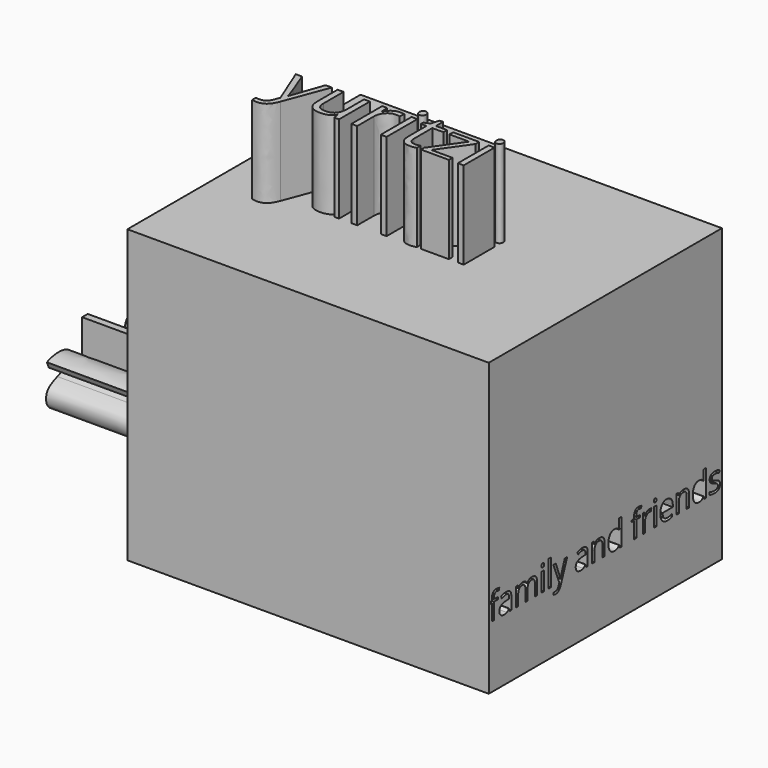
from build123d import *

# Parameters (mm, degrees)
F0_W         = 127
F0_H         = 127
F1_DEPTH     = 127
F2_TEXT_SIZE = 31.3097072419
F3_DEPTH     = 38.1
F4_TEXT_SIZE = 37.9493149618
F5_DEPTH     = 38.1
F6_TEXT_SIZE = 18.0097937116
F7_DEPTH     = 30.48
F8_W         = 127
F8_H         = 127
F8_W_2       = 1.2229891456
F8_H_2       = 8.0707857872
F8_H_3       = 11.4593376009
F9_DEPTH     = 30.48


# Not quite as in the source:
# - Text() gives the source's letters only with a copy of the font that has no kerning and outlines rounded to 1/6400 em; it was checked with that copy


with BuildPart() as f1:
    # F0 (on Front) → F1 (new body)
    with BuildSketch(Plane.XZ):
        with Locations((29.3806100488, 72.0371453315)):
            Rectangle(F0_W, F0_H)
    extrude(amount=F1_DEPTH)

    # F2 (on face) → F3 (join)
    with BuildSketch(Plane.XY.offset(135.5371453315)):
        with Locations((-15.0693899512, -75.8829892142)):
            Text('yuritzi', F2_TEXT_SIZE, font='Open Sans', text_align=(TextAlign.LEFT, TextAlign.BOTTOM))
    extrude(amount=F3_DEPTH)

    # F4 (on face) → F5 (join)
    with BuildSketch(Plane(origin=(-34.1193899512, 0, 0), x_dir=(0, -1, 0), z_dir=(-1, 0, 0))):
        with Locations((1.5054866672, 51.249936223)):
            Text('friends', F4_TEXT_SIZE, font='Open Sans', text_align=(TextAlign.LEFT, TextAlign.BOTTOM))
    extrude(amount=F5_DEPTH)

    # F6 (on face) → F7 (join)
    with BuildSketch(Plane(origin=(0, 0, 0), x_dir=(-1, 0, 0), z_dir=(0, 1, 0))):
        with Locations((-92.8806100488, 35.0644422385)):
            Text('happy holidays', F6_TEXT_SIZE, font='Open Sans', text_align=(TextAlign.LEFT, TextAlign.BOTTOM))
    extrude(amount=F7_DEPTH)

    # F8 (on face) → F9 (join)
    with BuildSketch(Plane.YZ.offset(92.8806100488)):
        with Locations((-63.5, 72.0371453315)):
            Rectangle(F8_W, F8_H)
        with BuildLine():
            Line((-114.7229798683, 35.6142357407), (-115.6302068838, 35.6142357407))
            Line((-115.6302068838, 35.6142357407), (-115.8729195658, 36.7641754382))
            Line((-115.8729195658, 36.7641754382), (-115.931830411, 36.7641754382))
            add(Edge.make_bspline(
                [(-115.931830411, 36.7641754382), (-116.5350774654, 36.0054037525), (-117.1347898692, 35.7355920817)],
                knots=[0, 0, 0, 1, 1, 1], degree=2))
            add(Edge.make_bspline(
                [(-117.1347898692, 35.7355920817), (-117.7345022729, 35.4657804109), (-118.634659987, 35.4657804109)],
                knots=[0, 0, 0, 1, 1, 1], degree=2))
            add(Edge.make_bspline(
                [(-118.634659987, 35.4657804109), (-119.8340847945, 35.4657804109), (-120.5150941646, 36.085522502)],
                knots=[0, 0, 0, 1, 1, 1], degree=2))
            add(Edge.make_bspline(
                [(-120.5150941646, 36.085522502), (-121.1961035347, 36.7052645931), (-121.1961035347, 37.8457785554)],
                knots=[0, 0, 0, 1, 1, 1], degree=2))
            add(Edge.make_bspline(
                [(-121.1961035347, 37.8457785554), (-121.1961035347, 40.2894004127), (-117.2867798497, 40.407222103)],
                knots=[0, 0, 0, 1, 1, 1], degree=2))
            Line((-117.2867798497, 40.407222103), (-115.9176918081, 40.4519943454))
            Line((-115.9176918081, 40.4519943454), (-115.9176918081, 40.9539147461))
            add(Edge.make_bspline(
                [(-115.9176918081, 40.9539147461), (-115.9176918081, 41.9035575701), (-116.3253548567, 42.355992861)],
                knots=[0, 0, 0, 1, 1, 1], degree=2))
            add(Edge.make_bspline(
                [(-116.3253548567, 42.355992861), (-116.7330179052, 42.8084281518), (-117.6331756193, 42.8084281518)],
                knots=[0, 0, 0, 1, 1, 1], degree=2))
            add(Edge.make_bspline(
                [(-117.6331756193, 42.8084281518), (-118.6417292884, 42.8084281518), (-119.9142035439, 42.1910424945)],
                knots=[0, 0, 0, 1, 1, 1], degree=2))
            Line((-119.9142035439, 42.1910424945), (-120.291232953, 43.1265467157))
            add(Edge.make_bspline(
                [(-120.291232953, 43.1265467157), (-119.6950551999, 43.4493781472), (-118.9845904073, 43.6331799841)],
                knots=[0, 0, 0, 1, 1, 1], degree=2))
            add(Edge.make_bspline(
                [(-118.9845904073, 43.6331799841), (-118.2741256146, 43.816981821), (-117.5577697375, 43.816981821)],
                knots=[0, 0, 0, 1, 1, 1], degree=2))
            add(Edge.make_bspline(
                [(-117.5577697375, 43.816981821), (-116.1156322479, 43.816981821), (-115.4193060581, 43.1772100425)],
                knots=[0, 0, 0, 1, 1, 1], degree=2))
            add(Edge.make_bspline(
                [(-115.4193060581, 43.1772100425), (-114.7229798683, 42.5374382641), (-114.7229798683, 41.1235779802)],
                knots=[0, 0, 0, 1, 1, 1], degree=2))
            Line((-114.7229798683, 41.1235779802), (-114.7229798683, 35.6142357407))
        make_face(mode=Mode.SUBTRACT)
        with BuildLine():
            Line((-100.6974858521, 35.6142357407), (-101.9181185639, 35.6142357407))
            Line((-101.9181185639, 35.6142357407), (-101.9181185639, 40.8643702615))
            add(Edge.make_bspline(
                [(-101.9181185639, 40.8643702615), (-101.9181185639, 41.8305081221), (-102.33049448, 42.3123988356)],
                knots=[0, 0, 0, 1, 1, 1], degree=2))
            add(Edge.make_bspline(
                [(-102.33049448, 42.3123988356), (-102.7428703961, 42.794289549), (-103.6123944707, 42.794289549)],
                knots=[0, 0, 0, 1, 1, 1], degree=2))
            add(Edge.make_bspline(
                [(-103.6123944707, 42.794289549), (-104.7529084331, 42.794289549), (-105.2984228593, 42.1392009508)],
                knots=[0, 0, 0, 1, 1, 1], degree=2))
            add(Edge.make_bspline(
                [(-105.2984228593, 42.1392009508), (-105.8439372855, 41.4841123526), (-105.8439372855, 40.1220936124)],
                knots=[0, 0, 0, 1, 1, 1], degree=2))
            Line((-105.8439372855, 40.1220936124), (-105.8439372855, 35.6142357407))
            Line((-105.8439372855, 35.6142357407), (-107.066926431, 35.6142357407))
            Line((-107.066926431, 35.6142357407), (-107.066926431, 40.8643702615))
            add(Edge.make_bspline(
                [(-107.066926431, 40.8643702615), (-107.066926431, 41.8305081221), (-107.4793023472, 42.3123988356)],
                knots=[0, 0, 0, 1, 1, 1], degree=2))
            add(Edge.make_bspline(
                [(-107.4793023472, 42.3123988356), (-107.8916782633, 42.794289549), (-108.7682716393, 42.794289549)],
                knots=[0, 0, 0, 1, 1, 1], degree=2))
            add(Edge.make_bspline(
                [(-108.7682716393, 42.794289549), (-109.9158549031, 42.794289549), (-110.4495871602, 42.1062108775)],
                knots=[0, 0, 0, 1, 1, 1], degree=2))
            add(Edge.make_bspline(
                [(-110.4495871602, 42.1062108775), (-110.9833194174, 41.418132206), (-110.9833194174, 39.8487472909)],
                knots=[0, 0, 0, 1, 1, 1], degree=2))
            Line((-110.9833194174, 39.8487472909), (-110.9833194174, 35.6142357407))
            Line((-110.9833194174, 35.6142357407), (-112.2063085629, 35.6142357407))
            Line((-112.2063085629, 35.6142357407), (-112.2063085629, 43.6850215278))
            Line((-112.2063085629, 43.6850215278), (-111.2118934966, 43.6850215278))
            Line((-111.2118934966, 43.6850215278), (-111.0139530569, 42.5798540726))
            Line((-111.0139530569, 42.5798540726), (-110.9550422117, 42.5798540726))
            add(Edge.make_bspline(
                [(-110.9550422117, 42.5798540726), (-110.6086464422, 43.1689625242), (-109.9783003989, 43.5012196909)],
                knots=[0, 0, 0, 1, 1, 1], degree=2))
            add(Edge.make_bspline(
                [(-109.9783003989, 43.5012196909), (-109.3479543557, 43.8334768576), (-108.5679747657, 43.8334768576)],
                knots=[0, 0, 0, 1, 1, 1], degree=2))
            add(Edge.make_bspline(
                [(-108.5679747657, 43.8334768576), (-106.6757584191, 43.8334768576), (-106.0937192689, 42.4620323823)],
                knots=[0, 0, 0, 1, 1, 1], degree=2))
            Line((-106.0937192689, 42.4620323823), (-106.0348084238, 42.4620323823))
            add(Edge.make_bspline(
                [(-106.0348084238, 42.4620323823), (-105.6742740514, 43.0959130762), (-104.9897300306, 43.4646949669)],
                knots=[0, 0, 0, 1, 1, 1], degree=2))
            add(Edge.make_bspline(
                [(-104.9897300306, 43.4646949669), (-104.3051860098, 43.8334768576), (-103.4285926338, 43.8334768576)],
                knots=[0, 0, 0, 1, 1, 1], degree=2))
            add(Edge.make_bspline(
                [(-103.4285926338, 43.8334768576), (-102.0595045923, 43.8334768576), (-101.3784952222, 43.1300813664)],
                knots=[0, 0, 0, 1, 1, 1], degree=2))
            add(Edge.make_bspline(
                [(-101.3784952222, 43.1300813664), (-100.6974858521, 42.4266858752), (-100.6974858521, 40.8785088643)],
                knots=[0, 0, 0, 1, 1, 1], degree=2))
            Line((-100.6974858521, 40.8785088643), (-100.6974858521, 35.6142357407))
        make_face(mode=Mode.SUBTRACT)
        with Locations((-97.5669635402, 39.6496286343)):
            Rectangle(F8_W_2, F8_H_2, mode=Mode.SUBTRACT)
        with BuildLine():
            Line((-88.5736339178, 35.5694634983), (-91.8302254384, 43.6850215278))
            Line((-91.8302254384, 43.6850215278), (-90.5176918081, 43.6850215278))
            Line((-90.5176918081, 43.6850215278), (-88.7503664533, 39.0829063038))
            add(Edge.make_bspline(
                [(-88.7503664533, 39.0829063038), (-88.1706837369, 37.5064520873), (-88.0292977085, 36.8065912467)],
                knots=[0, 0, 0, 1, 1, 1], degree=2))
            Line((-88.0292977085, 36.8065912467), (-87.9703868633, 36.8065912467))
            add(Edge.make_bspline(
                [(-87.9703868633, 36.8065912467), (-87.8761295111, 37.1836206558), (-87.5697931162, 38.0932041051)],
                knots=[0, 0, 0, 1, 1, 1], degree=2))
            add(Edge.make_bspline(
                [(-87.5697931162, 38.0932041051), (-87.2634567214, 39.0027875544), (-85.5691808145, 43.6850215278)],
                knots=[0, 0, 0, 1, 1, 1], degree=2))
            Line((-85.5691808145, 43.6850215278), (-84.2590036181, 43.6850215278))
            Line((-84.2590036181, 43.6850215278), (-87.7276741813, 34.4949296826))
            add(Edge.make_bspline(
                [(-87.7276741813, 34.4949296826), (-88.2437331849, 33.1329109424), (-88.9318118564, 32.5614757444)],
                knots=[0, 0, 0, 1, 1, 1], degree=2))
            add(Edge.make_bspline(
                [(-88.9318118564, 32.5614757444), (-89.6198905279, 31.9900405463), (-90.6213748956, 31.9900405463)],
                knots=[0, 0, 0, 1, 1, 1], degree=2))
            add(Edge.make_bspline(
                [(-90.6213748956, 31.9900405463), (-91.1822061416, 31.9900405463), (-91.7265423509, 32.1172879719)],
                knots=[0, 0, 0, 1, 1, 1], degree=2))
            Line((-91.7265423509, 32.1172879719), (-91.7265423509, 33.0952080015))
            add(Edge.make_bspline(
                [(-91.7265423509, 33.0952080015), (-91.3212357362, 33.0080199507), (-90.8216717692, 33.0080199507)],
                knots=[0, 0, 0, 1, 1, 1], degree=2))
            add(Edge.make_bspline(
                [(-90.8216717692, 33.0080199507), (-89.5609796827, 33.0080199507), (-89.0237127748, 34.4218802346)],
                knots=[0, 0, 0, 1, 1, 1], degree=2))
            Line((-89.0237127748, 34.4218802346), (-88.5736339178, 35.5694634983))
        make_face(mode=Mode.SUBTRACT)
        with BuildLine():
            Line((-73.1602003896, 35.6142357407), (-74.0674274051, 35.6142357407))
            Line((-74.0674274051, 35.6142357407), (-74.3101400872, 36.7641754382))
            Line((-74.3101400872, 36.7641754382), (-74.3690509324, 36.7641754382))
            add(Edge.make_bspline(
                [(-74.3690509324, 36.7641754382), (-74.9722979868, 36.0054037525), (-75.5720103906, 35.7355920817)],
                knots=[0, 0, 0, 1, 1, 1], degree=2))
            add(Edge.make_bspline(
                [(-75.5720103906, 35.7355920817), (-76.1717227943, 35.4657804109), (-77.0718805084, 35.4657804109)],
                knots=[0, 0, 0, 1, 1, 1], degree=2))
            add(Edge.make_bspline(
                [(-77.0718805084, 35.4657804109), (-78.2713053159, 35.4657804109), (-78.952314686, 36.085522502)],
                knots=[0, 0, 0, 1, 1, 1], degree=2))
            add(Edge.make_bspline(
                [(-78.952314686, 36.085522502), (-79.633324056, 36.7052645931), (-79.633324056, 37.8457785554)],
                knots=[0, 0, 0, 1, 1, 1], degree=2))
            add(Edge.make_bspline(
                [(-79.633324056, 37.8457785554), (-79.633324056, 40.2894004127), (-75.7240003711, 40.407222103)],
                knots=[0, 0, 0, 1, 1, 1], degree=2))
            Line((-75.7240003711, 40.407222103), (-74.3549123295, 40.4519943454))
            Line((-74.3549123295, 40.4519943454), (-74.3549123295, 40.9539147461))
            add(Edge.make_bspline(
                [(-74.3549123295, 40.9539147461), (-74.3549123295, 41.9035575701), (-74.762575378, 42.355992861)],
                knots=[0, 0, 0, 1, 1, 1], degree=2))
            add(Edge.make_bspline(
                [(-74.762575378, 42.355992861), (-75.1702384266, 42.8084281518), (-76.0703961406, 42.8084281518)],
                knots=[0, 0, 0, 1, 1, 1], degree=2))
            add(Edge.make_bspline(
                [(-76.0703961406, 42.8084281518), (-77.0789498098, 42.8084281518), (-78.3514240653, 42.1910424945)],
                knots=[0, 0, 0, 1, 1, 1], degree=2))
            Line((-78.3514240653, 42.1910424945), (-78.7284534743, 43.1265467157))
            add(Edge.make_bspline(
                [(-78.7284534743, 43.1265467157), (-78.1322757213, 43.4493781472), (-77.4218109287, 43.6331799841)],
                knots=[0, 0, 0, 1, 1, 1], degree=2))
            add(Edge.make_bspline(
                [(-77.4218109287, 43.6331799841), (-76.711346136, 43.816981821), (-75.9949902588, 43.816981821)],
                knots=[0, 0, 0, 1, 1, 1], degree=2))
            add(Edge.make_bspline(
                [(-75.9949902588, 43.816981821), (-74.5528527693, 43.816981821), (-73.8565265795, 43.1772100425)],
                knots=[0, 0, 0, 1, 1, 1], degree=2))
            add(Edge.make_bspline(
                [(-73.8565265795, 43.1772100425), (-73.1602003896, 42.5374382641), (-73.1602003896, 41.1235779802)],
                knots=[0, 0, 0, 1, 1, 1], degree=2))
            Line((-73.1602003896, 41.1235779802), (-73.1602003896, 35.6142357407))
        make_face(mode=Mode.SUBTRACT)
        with BuildLine():
            Line((-63.8970590964, 35.6142357407), (-65.120048242, 35.6142357407))
            Line((-65.120048242, 35.6142357407), (-65.120048242, 40.8360930558))
            add(Edge.make_bspline(
                [(-65.120048242, 40.8360930558), (-65.120048242, 41.8210823869), (-65.5689488821, 42.307685968)],
                knots=[0, 0, 0, 1, 1, 1], degree=2))
            add(Edge.make_bspline(
                [(-65.5689488821, 42.307685968), (-66.0178495222, 42.794289549), (-66.9769180815, 42.794289549)],
                knots=[0, 0, 0, 1, 1, 1], degree=2))
            add(Edge.make_bspline(
                [(-66.9769180815, 42.794289549), (-68.2423230355, 42.794289549), (-68.8314314872, 42.1097455282)],
                knots=[0, 0, 0, 1, 1, 1], degree=2))
            add(Edge.make_bspline(
                [(-68.8314314872, 42.1097455282), (-69.4205399388, 41.4252015074), (-69.4205399388, 39.8487472909)],
                knots=[0, 0, 0, 1, 1, 1], degree=2))
            Line((-69.4205399388, 39.8487472909), (-69.4205399388, 35.6142357407))
            Line((-69.4205399388, 35.6142357407), (-70.6435290843, 35.6142357407))
            Line((-70.6435290843, 35.6142357407), (-70.6435290843, 43.6850215278))
            Line((-70.6435290843, 43.6850215278), (-69.649114018, 43.6850215278))
            Line((-69.649114018, 43.6850215278), (-69.4511735783, 42.5798540726))
            Line((-69.4511735783, 42.5798540726), (-69.3922627331, 42.5798540726))
            add(Edge.make_bspline(
                [(-69.3922627331, 42.5798540726), (-69.0152333241, 43.1760318256), (-68.3377586047, 43.5047543416)],
                knots=[0, 0, 0, 1, 1, 1], degree=2))
            add(Edge.make_bspline(
                [(-68.3377586047, 43.5047543416), (-67.6602838853, 43.8334768576), (-66.8284627516, 43.8334768576)],
                knots=[0, 0, 0, 1, 1, 1], degree=2))
            add(Edge.make_bspline(
                [(-66.8284627516, 43.8334768576), (-65.3698302254, 43.8334768576), (-64.6334446609, 43.1300813664)],
                knots=[0, 0, 0, 1, 1, 1], degree=2))
            add(Edge.make_bspline(
                [(-64.6334446609, 43.1300813664), (-63.8970590964, 42.4266858752), (-63.8970590964, 40.8785088643)],
                knots=[0, 0, 0, 1, 1, 1], degree=2))
            Line((-63.8970590964, 40.8785088643), (-63.8970590964, 35.6142357407))
        make_face(mode=Mode.SUBTRACT)
        with BuildLine():
            Line((-122.0656276092, 43.6850215278), (-122.0656276092, 42.7353787038))
            Line((-122.0656276092, 42.7353787038), (-124.1204378885, 42.7353787038))
            Line((-124.1204378885, 42.7353787038), (-124.1204378885, 35.6142357407))
            Line((-124.1204378885, 35.6142357407), (-125.343427034, 35.6142357407))
            Line((-125.343427034, 35.6142357407), (-125.343427034, 42.7353787038))
            Line((-125.343427034, 42.7353787038), (-126.7855645236, 42.7353787038))
            Line((-126.7855645236, 42.7353787038), (-126.7855645236, 43.2867842145))
            Line((-126.7855645236, 43.2867842145), (-125.343427034, 43.7297937702))
            Line((-125.343427034, 43.7297937702), (-125.343427034, 44.1775161934))
            add(Edge.make_bspline(
                [(-125.343427034, 44.1775161934), (-125.343427034, 47.153692091), (-122.7442805455, 47.153692091)],
                knots=[0, 0, 0, 1, 1, 1], degree=2))
            add(Edge.make_bspline(
                [(-122.7442805455, 47.153692091), (-122.1033305501, 47.153692091), (-121.240875777, 46.8968408061)],
                knots=[0, 0, 0, 1, 1, 1], degree=2))
            Line((-121.240875777, 46.8968408061), (-121.5589943408, 45.9165643426))
            add(Edge.make_bspline(
                [(-121.5589943408, 45.9165643426), (-122.2659244828, 46.1451384218), (-122.7654884498, 46.1451384218)],
                knots=[0, 0, 0, 1, 1, 1], degree=2))
            add(Edge.make_bspline(
                [(-122.7654884498, 46.1451384218), (-123.4582799889, 46.1451384218), (-123.7893589387, 45.6844556126)],
                knots=[0, 0, 0, 1, 1, 1], degree=2))
            add(Edge.make_bspline(
                [(-123.7893589387, 45.6844556126), (-124.1204378885, 45.2237728035), (-124.1204378885, 44.2081498329)],
                knots=[0, 0, 0, 1, 1, 1], degree=2))
            Line((-124.1204378885, 44.2081498329), (-124.1204378885, 43.6850215278))
            Line((-124.1204378885, 43.6850215278), (-122.0656276092, 43.6850215278))
        make_face(mode=Mode.SUBTRACT)
        with BuildLine():
            add(Edge.make_bspline(
                [(-98.0759532424, 45.2567628768), (-98.2821412005, 45.4594161841), (-98.2821412005, 45.8717921002)],
                knots=[0, 0, 0, 1, 1, 1], degree=2))
            add(Edge.make_bspline(
                [(-98.2821412005, 45.8717921002), (-98.2821412005, 46.2912373178), (-98.0759532424, 46.4868213237)],
                knots=[0, 0, 0, 1, 1, 1], degree=2))
            add(Edge.make_bspline(
                [(-98.0759532424, 46.4868213237), (-97.8697652843, 46.6824053297), (-97.5587160219, 46.6824053297)],
                knots=[0, 0, 0, 1, 1, 1], degree=2))
            add(Edge.make_bspline(
                [(-97.5587160219, 46.6824053297), (-97.2641617961, 46.6824053297), (-97.0509045366, 46.483286673)],
                knots=[0, 0, 0, 1, 1, 1], degree=2))
            add(Edge.make_bspline(
                [(-97.0509045366, 46.483286673), (-96.8376472771, 46.2841680164), (-96.8376472771, 45.8717921002)],
                knots=[0, 0, 0, 1, 1, 1], degree=2))
            add(Edge.make_bspline(
                [(-96.8376472771, 45.8717921002), (-96.8376472771, 45.4594161841), (-97.0509045366, 45.2567628768)],
                knots=[0, 0, 0, 1, 1, 1], degree=2))
            add(Edge.make_bspline(
                [(-97.0509045366, 45.2567628768), (-97.2641617961, 45.0541095694), (-97.5587160219, 45.0541095694)],
                knots=[0, 0, 0, 1, 1, 1], degree=2))
            add(Edge.make_bspline(
                [(-97.5587160219, 45.0541095694), (-97.8697652843, 45.0541095694), (-98.0759532424, 45.2567628768)],
                knots=[0, 0, 0, 1, 1, 1], degree=2))
        make_face(mode=Mode.SUBTRACT)
        with Locations((-93.7518972075, 41.3439045411)):
            Rectangle(F8_W_2, F8_H_3, mode=Mode.SUBTRACT)
        with BuildLine():
            add(Edge.make_bspline(
                [(-40.8252156972, 43.4057841218), (-40.1913350032, 43.8334768576), (-39.4325633176, 43.8334768576)],
                knots=[0, 0, 0, 1, 1, 1], degree=2))
            add(Edge.make_bspline(
                [(-39.4325633176, 43.8334768576), (-38.8952964097, 43.8334768576), (-38.4687818907, 43.743932373)],
                knots=[0, 0, 0, 1, 1, 1], degree=2))
            Line((-38.4687818907, 43.743932373), (-38.6384451248, 42.6104877121))
            add(Edge.make_bspline(
                [(-38.6384451248, 42.6104877121), (-39.1380090918, 42.721240101), (-39.5221078022, 42.721240101)],
                knots=[0, 0, 0, 1, 1, 1], degree=2))
            add(Edge.make_bspline(
                [(-39.5221078022, 42.721240101), (-40.5023842657, 42.721240101), (-41.1975322386, 41.9259436913)],
                knots=[0, 0, 0, 1, 1, 1], degree=2))
            add(Edge.make_bspline(
                [(-41.1975322386, 41.9259436913), (-41.8926802115, 41.1306472816), (-41.8926802115, 39.945361077)],
                knots=[0, 0, 0, 1, 1, 1], degree=2))
            Line((-41.8926802115, 39.945361077), (-41.8926802115, 35.6142357407))
            Line((-41.8926802115, 35.6142357407), (-43.1156693571, 35.6142357407))
            Line((-43.1156693571, 35.6142357407), (-43.1156693571, 43.6850215278))
            Line((-43.1156693571, 43.6850215278), (-42.1071156879, 43.6850215278))
            Line((-42.1071156879, 43.6850215278), (-41.9657296595, 42.1910424945))
            Line((-41.9657296595, 42.1910424945), (-41.9068188144, 42.1910424945))
            add(Edge.make_bspline(
                [(-41.9068188144, 42.1910424945), (-41.4590963911, 42.9780913859), (-40.8252156972, 43.4057841218)],
                knots=[0, 0, 0, 1, 1, 1], degree=2))
        make_face(mode=Mode.SUBTRACT)
        with Locations((-36.346813248, 39.6496286343)):
            Rectangle(F8_W_2, F8_H_2, mode=Mode.SUBTRACT)
        with BuildLine():
            add(Edge.make_bspline(
                [(-28.3384729567, 35.5883149688), (-28.9157992393, 35.4657804109), (-29.7334817701, 35.4657804109)],
                knots=[0, 0, 0, 1, 1, 1], degree=2))
            add(Edge.make_bspline(
                [(-29.7334817701, 35.4657804109), (-31.5220150292, 35.4657804109), (-32.5576676872, 36.5568092633)],
                knots=[0, 0, 0, 1, 1, 1], degree=2))
            add(Edge.make_bspline(
                [(-32.5576676872, 36.5568092633), (-33.5933203451, 37.6478381156), (-33.5933203451, 39.5824702708)],
                knots=[0, 0, 0, 1, 1, 1], degree=2))
            add(Edge.make_bspline(
                [(-33.5933203451, 39.5824702708), (-33.5933203451, 41.5359538963), (-32.6318953521, 42.684715377)],
                knots=[0, 0, 0, 1, 1, 1], degree=2))
            add(Edge.make_bspline(
                [(-32.6318953521, 42.684715377), (-31.670470359, 43.8334768576), (-30.0492439002, 43.8334768576)],
                knots=[0, 0, 0, 1, 1, 1], degree=2))
            add(Edge.make_bspline(
                [(-30.0492439002, 43.8334768576), (-28.5340569626, 43.8334768576), (-27.6503942852, 42.8355271406)],
                knots=[0, 0, 0, 1, 1, 1], degree=2))
            add(Edge.make_bspline(
                [(-27.6503942852, 42.8355271406), (-26.7667316078, 41.8375774236), (-26.7667316078, 40.2022123619)],
                knots=[0, 0, 0, 1, 1, 1], degree=2))
            Line((-26.7667316078, 40.2022123619), (-26.7667316078, 39.4293020733))
            Line((-26.7667316078, 39.4293020733), (-32.3255589572, 39.4293020733))
            add(Edge.make_bspline(
                [(-32.3255589572, 39.4293020733), (-32.2878560163, 38.008372488), (-31.6068466463, 37.2719869235)],
                knots=[0, 0, 0, 1, 1, 1], degree=2))
            add(Edge.make_bspline(
                [(-31.6068466463, 37.2719869235), (-30.9258372762, 36.535601359), (-29.6887095278, 36.535601359)],
                knots=[0, 0, 0, 1, 1, 1], degree=2))
            add(Edge.make_bspline(
                [(-29.6887095278, 36.535601359), (-28.3856016328, 36.535601359), (-27.1131273773, 37.0799375683)],
                knots=[0, 0, 0, 1, 1, 1], degree=2))
            Line((-27.1131273773, 37.0799375683), (-27.1131273773, 35.9889087159))
            add(Edge.make_bspline(
                [(-27.1131273773, 35.9889087159), (-27.7611466741, 35.7108495267), (-28.3384729567, 35.5883149688)],
                knots=[0, 0, 0, 1, 1, 1], degree=2))
        make_face(mode=Mode.SUBTRACT)
        with BuildLine():
            Line((-17.9348177011, 35.6142357407), (-19.1578068466, 35.6142357407))
            Line((-19.1578068466, 35.6142357407), (-19.1578068466, 40.8360930558))
            add(Edge.make_bspline(
                [(-19.1578068466, 40.8360930558), (-19.1578068466, 41.8210823869), (-19.6067074868, 42.307685968)],
                knots=[0, 0, 0, 1, 1, 1], degree=2))
            add(Edge.make_bspline(
                [(-19.6067074868, 42.307685968), (-20.0556081269, 42.794289549), (-21.0146766861, 42.794289549)],
                knots=[0, 0, 0, 1, 1, 1], degree=2))
            add(Edge.make_bspline(
                [(-21.0146766861, 42.794289549), (-22.2800816402, 42.794289549), (-22.8691900918, 42.1097455282)],
                knots=[0, 0, 0, 1, 1, 1], degree=2))
            add(Edge.make_bspline(
                [(-22.8691900918, 42.1097455282), (-23.4582985435, 41.4252015074), (-23.4582985435, 39.8487472909)],
                knots=[0, 0, 0, 1, 1, 1], degree=2))
            Line((-23.4582985435, 39.8487472909), (-23.4582985435, 35.6142357407))
            Line((-23.4582985435, 35.6142357407), (-24.681287689, 35.6142357407))
            Line((-24.681287689, 35.6142357407), (-24.681287689, 43.6850215278))
            Line((-24.681287689, 43.6850215278), (-23.6868726227, 43.6850215278))
            Line((-23.6868726227, 43.6850215278), (-23.4889321829, 42.5798540726))
            Line((-23.4889321829, 42.5798540726), (-23.4300213378, 42.5798540726))
            add(Edge.make_bspline(
                [(-23.4300213378, 42.5798540726), (-23.0529919288, 43.1760318256), (-22.3755172094, 43.5047543416)],
                knots=[0, 0, 0, 1, 1, 1], degree=2))
            add(Edge.make_bspline(
                [(-22.3755172094, 43.5047543416), (-21.69804249, 43.8334768576), (-20.8662213563, 43.8334768576)],
                knots=[0, 0, 0, 1, 1, 1], degree=2))
            add(Edge.make_bspline(
                [(-20.8662213563, 43.8334768576), (-19.4075888301, 43.8334768576), (-18.6712032656, 43.1300813664)],
                knots=[0, 0, 0, 1, 1, 1], degree=2))
            add(Edge.make_bspline(
                [(-18.6712032656, 43.1300813664), (-17.9348177011, 42.4266858752), (-17.9348177011, 40.8785088643)],
                knots=[0, 0, 0, 1, 1, 1], degree=2))
            Line((-17.9348177011, 40.8785088643), (-17.9348177011, 35.6142357407))
        make_face(mode=Mode.SUBTRACT)
        with BuildLine():
            add(Edge.make_bspline(
                [(-1.4821968643, 39.1488864504), (-0.9779200297, 38.6186888439), (-0.9779200297, 37.8151449159)],
                knots=[0, 0, 0, 1, 1, 1], degree=2))
            add(Edge.make_bspline(
                [(-0.9779200297, 37.8151449159), (-0.9779200297, 36.6887695564), (-1.8168104648, 36.0772749836)],
                knots=[0, 0, 0, 1, 1, 1], degree=2))
            add(Edge.make_bspline(
                [(-1.8168104648, 36.0772749836), (-2.6557008999, 35.4657804109), (-4.1732442713, 35.4657804109)],
                knots=[0, 0, 0, 1, 1, 1], degree=2))
            add(Edge.make_bspline(
                [(-4.1732442713, 35.4657804109), (-5.7779756935, 35.4657804109), (-6.6757769737, 35.9747701131)],
                knots=[0, 0, 0, 1, 1, 1], degree=2))
            Line((-6.6757769737, 35.9747701131), (-6.6757769737, 37.108214774))
            add(Edge.make_bspline(
                [(-6.6757769737, 37.108214774), (-6.0937378235, 36.8136605482), (-5.4280452732, 36.645175531)],
                knots=[0, 0, 0, 1, 1, 1], degree=2))
            add(Edge.make_bspline(
                [(-5.4280452732, 36.645175531), (-4.7623527229, 36.4766905138), (-4.1426106318, 36.4766905138)],
                knots=[0, 0, 0, 1, 1, 1], degree=2))
            add(Edge.make_bspline(
                [(-4.1426106318, 36.4766905138), (-3.1858985064, 36.4766905138), (-2.6710177196, 36.7818486918)],
                knots=[0, 0, 0, 1, 1, 1], degree=2))
            add(Edge.make_bspline(
                [(-2.6710177196, 36.7818486918), (-2.1561369329, 37.0870068697), (-2.1561369329, 37.7138182622)],
                knots=[0, 0, 0, 1, 1, 1], degree=2))
            add(Edge.make_bspline(
                [(-2.1561369329, 37.7138182622), (-2.1561369329, 38.1851050235), (-2.5637999814, 38.519718624)],
                knots=[0, 0, 0, 1, 1, 1], degree=2))
            add(Edge.make_bspline(
                [(-2.5637999814, 38.519718624), (-2.97146303, 38.8543322246), (-4.1591056684, 39.311480383)],
                knots=[0, 0, 0, 1, 1, 1], degree=2))
            add(Edge.make_bspline(
                [(-4.1591056684, 39.311480383), (-5.2854810279, 39.7309256006), (-5.7603024399, 40.0443312968)],
                knots=[0, 0, 0, 1, 1, 1], degree=2))
            add(Edge.make_bspline(
                [(-5.7603024399, 40.0443312968), (-6.2351238519, 40.3577369931), (-6.4672325819, 40.7547960895)],
                knots=[0, 0, 0, 1, 1, 1], degree=2))
            add(Edge.make_bspline(
                [(-6.4672325819, 40.7547960895), (-6.6993413118, 41.1518551859), (-6.6993413118, 41.7032606966)],
                knots=[0, 0, 0, 1, 1, 1], degree=2))
            add(Edge.make_bspline(
                [(-6.6993413118, 41.7032606966), (-6.6993413118, 42.6906064615), (-5.8957973838, 43.2620416596)],
                knots=[0, 0, 0, 1, 1, 1], degree=2))
            add(Edge.make_bspline(
                [(-5.8957973838, 43.2620416596), (-5.0922534558, 43.8334768576), (-3.6948882086, 43.8334768576)],
                knots=[0, 0, 0, 1, 1, 1], degree=2))
            add(Edge.make_bspline(
                [(-3.6948882086, 43.8334768576), (-2.3917803136, 43.8334768576), (-1.1452268299, 43.3032792512)],
                knots=[0, 0, 0, 1, 1, 1], degree=2))
            Line((-1.1452268299, 43.3032792512), (-1.5811670841, 42.3088641849))
            add(Edge.make_bspline(
                [(-1.5811670841, 42.3088641849), (-2.7947304945, 42.8084281518), (-3.7820762594, 42.8084281518)],
                knots=[0, 0, 0, 1, 1, 1], degree=2))
            add(Edge.make_bspline(
                [(-3.7820762594, 42.8084281518), (-4.651600334, 42.8084281518), (-5.0934316727, 42.5362600472)],
                knots=[0, 0, 0, 1, 1, 1], degree=2))
            add(Edge.make_bspline(
                [(-5.0934316727, 42.5362600472), (-5.5352630114, 42.2640919425), (-5.5352630114, 41.7857358798)],
                knots=[0, 0, 0, 1, 1, 1], degree=2))
            add(Edge.make_bspline(
                [(-5.5352630114, 41.7857358798), (-5.5352630114, 41.4605480145), (-5.3691344281, 41.2331521522)],
                knots=[0, 0, 0, 1, 1, 1], degree=2))
            add(Edge.make_bspline(
                [(-5.3691344281, 41.2331521522), (-5.2030058447, 41.0057562899), (-4.8354021709, 40.7995683318)],
                knots=[0, 0, 0, 1, 1, 1], degree=2))
            add(Edge.make_bspline(
                [(-4.8354021709, 40.7995683318), (-4.4677984971, 40.5933803737), (-3.421541887, 40.2022123619)],
                knots=[0, 0, 0, 1, 1, 1], degree=2))
            add(Edge.make_bspline(
                [(-3.421541887, 40.2022123619), (-1.9864736989, 39.6790840568), (-1.4821968643, 39.1488864504)],
                knots=[0, 0, 0, 1, 1, 1], degree=2))
        make_face(mode=Mode.SUBTRACT)
        with BuildLine():
            Line((-55.732015957, 35.6142357407), (-55.8946098896, 36.6958388578))
            Line((-55.8946098896, 36.6958388578), (-55.9605900362, 36.6958388578))
            add(Edge.make_bspline(
                [(-55.9605900362, 36.6958388578), (-56.8065497727, 35.4657804109), (-58.4937563781, 35.4657804109)],
                knots=[0, 0, 0, 1, 1, 1], degree=2))
            add(Edge.make_bspline(
                [(-58.4937563781, 35.4657804109), (-60.0772798961, 35.4657804109), (-60.9574079228, 36.5485617449)],
                knots=[0, 0, 0, 1, 1, 1], degree=2))
            add(Edge.make_bspline(
                [(-60.9574079228, 36.5485617449), (-61.8375359495, 37.631343079), (-61.8375359495, 39.6272425131)],
                knots=[0, 0, 0, 1, 1, 1], degree=2))
            add(Edge.make_bspline(
                [(-61.8375359495, 39.6272425131), (-61.8375359495, 41.6231419472), (-60.9538732721, 42.7283094024)],
                knots=[0, 0, 0, 1, 1, 1], degree=2))
            add(Edge.make_bspline(
                [(-60.9538732721, 42.7283094024), (-60.0702105947, 43.8334768576), (-58.4937563781, 43.8334768576)],
                knots=[0, 0, 0, 1, 1, 1], degree=2))
            add(Edge.make_bspline(
                [(-58.4937563781, 43.8334768576), (-56.851322015, 43.8334768576), (-55.974728639, 42.6387649178)],
                knots=[0, 0, 0, 1, 1, 1], degree=2))
            Line((-55.974728639, 42.6387649178), (-55.878114853, 42.6387649178))
            Line((-55.878114853, 42.6387649178), (-55.9299563967, 43.220804068))
            Line((-55.9299563967, 43.220804068), (-55.9605900362, 43.7887046153))
            Line((-55.9605900362, 43.7887046153), (-55.9605900362, 47.0735733416))
            Line((-55.9605900362, 47.0735733416), (-54.7376008906, 47.0735733416))
            Line((-54.7376008906, 47.0735733416), (-54.7376008906, 35.6142357407))
            Line((-54.7376008906, 35.6142357407), (-55.732015957, 35.6142357407))
        make_face(mode=Mode.SUBTRACT)
        with BuildLine():
            Line((-44.5884404861, 43.6850215278), (-44.5884404861, 42.7353787038))
            Line((-44.5884404861, 42.7353787038), (-46.6432507654, 42.7353787038))
            Line((-46.6432507654, 42.7353787038), (-46.6432507654, 35.6142357407))
            Line((-46.6432507654, 35.6142357407), (-47.8662399109, 35.6142357407))
            Line((-47.8662399109, 35.6142357407), (-47.8662399109, 42.7353787038))
            Line((-47.8662399109, 42.7353787038), (-49.3083774005, 42.7353787038))
            Line((-49.3083774005, 42.7353787038), (-49.3083774005, 43.2867842145))
            Line((-49.3083774005, 43.2867842145), (-47.8662399109, 43.7297937702))
            Line((-47.8662399109, 43.7297937702), (-47.8662399109, 44.1775161934))
            add(Edge.make_bspline(
                [(-47.8662399109, 44.1775161934), (-47.8662399109, 47.153692091), (-45.2670934224, 47.153692091)],
                knots=[0, 0, 0, 1, 1, 1], degree=2))
            add(Edge.make_bspline(
                [(-45.2670934224, 47.153692091), (-44.626143427, 47.153692091), (-43.7636886539, 46.8968408061)],
                knots=[0, 0, 0, 1, 1, 1], degree=2))
            Line((-43.7636886539, 46.8968408061), (-44.0818072177, 45.9165643426))
            add(Edge.make_bspline(
                [(-44.0818072177, 45.9165643426), (-44.7887373597, 46.1451384218), (-45.2883013267, 46.1451384218)],
                knots=[0, 0, 0, 1, 1, 1], degree=2))
            add(Edge.make_bspline(
                [(-45.2883013267, 46.1451384218), (-45.9810928658, 46.1451384218), (-46.3121718156, 45.6844556126)],
                knots=[0, 0, 0, 1, 1, 1], degree=2))
            add(Edge.make_bspline(
                [(-46.3121718156, 45.6844556126), (-46.6432507654, 45.2237728035), (-46.6432507654, 44.2081498329)],
                knots=[0, 0, 0, 1, 1, 1], degree=2))
            Line((-46.6432507654, 44.2081498329), (-46.6432507654, 43.6850215278))
            Line((-46.6432507654, 43.6850215278), (-44.5884404861, 43.6850215278))
        make_face(mode=Mode.SUBTRACT)
        with BuildLine():
            add(Edge.make_bspline(
                [(-36.8558029502, 45.2567628768), (-37.0619909082, 45.4594161841), (-37.0619909082, 45.8717921002)],
                knots=[0, 0, 0, 1, 1, 1], degree=2))
            add(Edge.make_bspline(
                [(-37.0619909082, 45.8717921002), (-37.0619909082, 46.2912373178), (-36.8558029502, 46.4868213237)],
                knots=[0, 0, 0, 1, 1, 1], degree=2))
            add(Edge.make_bspline(
                [(-36.8558029502, 46.4868213237), (-36.6496149921, 46.6824053297), (-36.3385657297, 46.6824053297)],
                knots=[0, 0, 0, 1, 1, 1], degree=2))
            add(Edge.make_bspline(
                [(-36.3385657297, 46.6824053297), (-36.0440115039, 46.6824053297), (-35.8307542444, 46.483286673)],
                knots=[0, 0, 0, 1, 1, 1], degree=2))
            add(Edge.make_bspline(
                [(-35.8307542444, 46.483286673), (-35.6174969849, 46.2841680164), (-35.6174969849, 45.8717921002)],
                knots=[0, 0, 0, 1, 1, 1], degree=2))
            add(Edge.make_bspline(
                [(-35.6174969849, 45.8717921002), (-35.6174969849, 45.4594161841), (-35.8307542444, 45.2567628768)],
                knots=[0, 0, 0, 1, 1, 1], degree=2))
            add(Edge.make_bspline(
                [(-35.8307542444, 45.2567628768), (-36.0440115039, 45.0541095694), (-36.3385657297, 45.0541095694)],
                knots=[0, 0, 0, 1, 1, 1], degree=2))
            add(Edge.make_bspline(
                [(-36.3385657297, 45.0541095694), (-36.6496149921, 45.0541095694), (-36.8558029502, 45.2567628768)],
                knots=[0, 0, 0, 1, 1, 1], degree=2))
        make_face(mode=Mode.SUBTRACT)
        with BuildLine():
            Line((-9.7697745616, 35.6142357407), (-9.9323684943, 36.6958388578))
            Line((-9.9323684943, 36.6958388578), (-9.9983486409, 36.6958388578))
            add(Edge.make_bspline(
                [(-9.9983486409, 36.6958388578), (-10.8443083774, 35.4657804109), (-12.5315149828, 35.4657804109)],
                knots=[0, 0, 0, 1, 1, 1], degree=2))
            add(Edge.make_bspline(
                [(-12.5315149828, 35.4657804109), (-14.1150385008, 35.4657804109), (-14.9951665275, 36.5485617449)],
                knots=[0, 0, 0, 1, 1, 1], degree=2))
            add(Edge.make_bspline(
                [(-14.9951665275, 36.5485617449), (-15.8752945542, 37.631343079), (-15.8752945542, 39.6272425131)],
                knots=[0, 0, 0, 1, 1, 1], degree=2))
            add(Edge.make_bspline(
                [(-15.8752945542, 39.6272425131), (-15.8752945542, 41.6231419472), (-14.9916318768, 42.7283094024)],
                knots=[0, 0, 0, 1, 1, 1], degree=2))
            add(Edge.make_bspline(
                [(-14.9916318768, 42.7283094024), (-14.1079691994, 43.8334768576), (-12.5315149828, 43.8334768576)],
                knots=[0, 0, 0, 1, 1, 1], degree=2))
            add(Edge.make_bspline(
                [(-12.5315149828, 43.8334768576), (-10.8890806197, 43.8334768576), (-10.0124872437, 42.6387649178)],
                knots=[0, 0, 0, 1, 1, 1], degree=2))
            Line((-10.0124872437, 42.6387649178), (-9.9158734576, 42.6387649178))
            Line((-9.9158734576, 42.6387649178), (-9.9677150014, 43.220804068))
            Line((-9.9677150014, 43.220804068), (-9.9983486409, 43.7887046153))
            Line((-9.9983486409, 43.7887046153), (-9.9983486409, 47.0735733416))
            Line((-9.9983486409, 47.0735733416), (-8.7753594953, 47.0735733416))
            Line((-8.7753594953, 47.0735733416), (-8.7753594953, 35.6142357407))
            Line((-8.7753594953, 35.6142357407), (-9.7697745616, 35.6142357407))
        make_face(mode=Mode.SUBTRACT)
    extrude(amount=F9_DEPTH)


solid = f1.part
